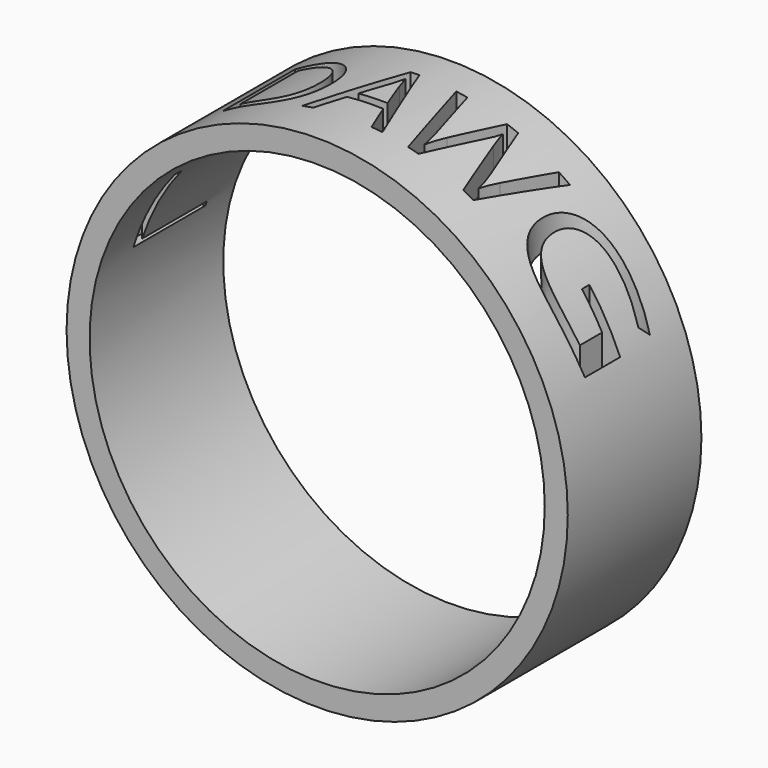
from build123d import *

# Parameters (mm, degrees)
F0_R         = 38.1
F1_DEPTH     = 25.4
F2_R         = 34.59949842
F3_DEPTH     = 25.4
F5_TEXT_SIZE = 19.2247712726
F6_DEPTH     = 38.1


# Not quite as in the source:
# - Text() gives the source's letters only with a copy of the font that has no kerning and outlines rounded to 1/6400 em; it was checked with that copy


with BuildPart() as f1:
    # F0 (on Front) → F1 (new body)
    with BuildSketch(Plane.XZ):
        with Locations((-4.7296555713, 17.3420701176)):
            Circle(F0_R)
    extrude(amount=F1_DEPTH)

    # F2 (on face) → F3 (cut)
    with BuildSketch(Plane.XZ.offset(25.4)):
        with Locations((-4.7296555713, 17.3420701176)):
            Circle(F2_R)
    extrude(amount=-F3_DEPTH, mode=Mode.SUBTRACT)

    # F5 (on offset) → F6 (cut)
    with BuildSketch(Plane.XY.offset(65.532)):
        with Locations((-41.1060545594, -18.9800416119)):
            Text('L DAWG', F5_TEXT_SIZE, font='Open Sans', text_align=(TextAlign.LEFT, TextAlign.BOTTOM))
    extrude(amount=-F6_DEPTH, mode=Mode.SUBTRACT)


solid = f1.part
